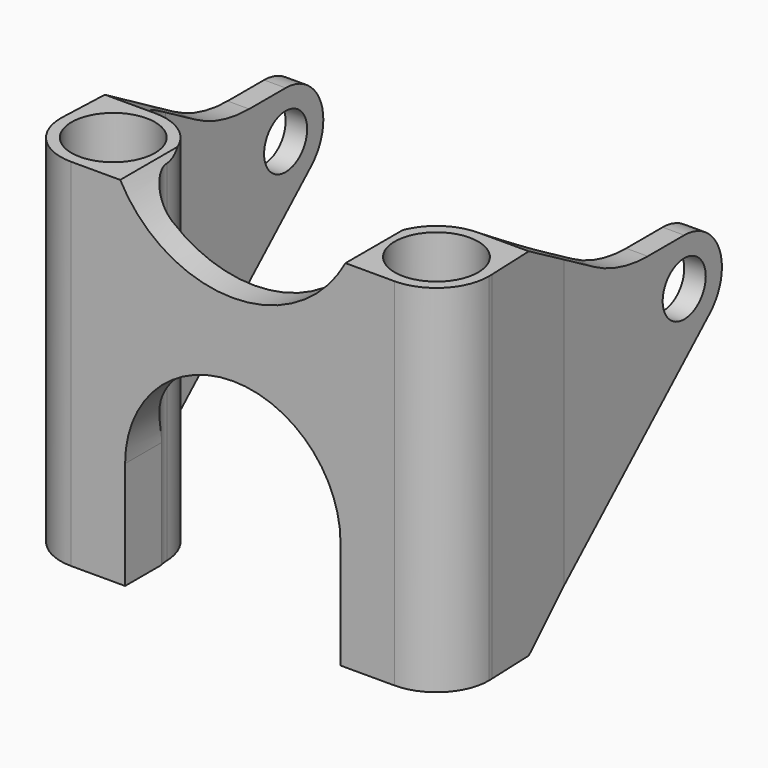
from build123d import *

# Parameters (mm, degrees)
F0_R          = 3.1
F1_DEPTH      = 35
F2_R          = 2
F3_DEPTH      = 31.501
F3_DEPTH_BACK = 0.301
F5_DEPTH      = 25.901


# Not quite as in the source:
# - a feature names something its author has since deleted; it is built from what else it names


with BuildPart() as f1:
    # F0 (on Top) → F1 (new body)
    with BuildSketch(Plane.XY):
        with BuildLine():
            ThreePointArc((-27.9, 0), (-26.7577164466, -2.7577164466), (-24, -3.9))
            ThreePointArc((-24, -3.9), (-21.2422835534, -2.7577164466), (-20.1, 0))
            ThreePointArc((-20.1, 0), (-21.2422835534, 2.7577164466), (-24, 3.9))
            ThreePointArc((-24, 3.9), (-26.643179735, 2.8676821456), (-27.8870765814, 0.3172312247))
            Line((-27.8870765814, 0.3172312247), (-27.9, 0))
        make_face()
        with Locations((-24, 0)):
            Circle(F0_R, mode=Mode.SUBTRACT)
        with BuildLine():
            Line((-27.6, 7.3641016151), (-27.8870765814, 0.3172312247))
            ThreePointArc((-27.8870765814, 0.3172312247), (-26.643179735, 2.8676821456), (-24, 3.9))
            ThreePointArc((-24, 3.9), (-25.4641016151, 5.3641016151), (-26, 7.3641016151))
            Line((-26, 7.3641016151), (-26, 22))
            Line((-26, 22), (-27.6, 22))
            Line((-27.6, 22), (-27.6, 7.3641016151))
        make_face()
        with BuildLine():
            ThreePointArc((0, -3.9), (-2.7577164466, -2.7577164466), (-3.9, 0))
            Line((-3.9, 0), (-3.9, 0.1))
            ThreePointArc((-3.9, 0.1), (-4.4857864376, -1.3142135624), (-5.9, -1.9))
            Line((-5.9, -1.9), (-18.1, -1.9))
            ThreePointArc((-18.1, -1.9), (-19.5142135624, -1.3142135624), (-20.1, 0.1))
            Line((-20.1, 0.1), (-20.1, 0))
            ThreePointArc((-20.1, 0), (-21.2422835534, -2.7577164466), (-24, -3.9))
            Line((-24, -3.9), (0, -3.9))
        make_face()
        with BuildLine():
            Line((3.9, 0), (3.8870765814, 0.3172312247))
            ThreePointArc((3.8870765814, 0.3172312247), (2.643179735, 2.8676821456), (0, 3.9))
            ThreePointArc((0, 3.9), (-2.7577164466, 2.7577164466), (-3.9, 0))
            ThreePointArc((-3.9, 0), (-2.7577164466, -2.7577164466), (0, -3.9))
            ThreePointArc((0, -3.9), (2.7577164466, -2.7577164466), (3.9, 0))
        make_face()
        Circle(F0_R, mode=Mode.SUBTRACT)
        with BuildLine():
            Line((3.6, 7.3641016151), (3.6, 22))
            Line((3.6, 22), (2, 22))
            Line((2, 22), (2, 7.3641016151))
            ThreePointArc((2, 7.3641016151), (1.4641016151, 5.3641016151), (0, 3.9))
            ThreePointArc((0, 3.9), (2.643179735, 2.8676821456), (3.8870765814, 0.3172312247))
            Line((3.8870765814, 0.3172312247), (3.6, 7.3641016151))
        make_face()
    extrude(amount=F1_DEPTH)

    # F2 (on face) → F3 (cut, two sides)
    with BuildSketch(Plane.YZ.offset(3.6)) as f3_sk:
        with BuildLine():
            ThreePointArc((18.5, 21.5), (20.9748737342, 20.4748737342), (22, 18))
            Line((22, 18), (22, 35))
            Line((22, 35), (7.3641016151, 35))
            Line((7.3641016151, 35), (7.3641016151, 24.4293139302))
            Line((7.3641016151, 24.4293139302), (10.1173140978, 22.8397459622))
            ThreePointArc((10.1173140978, 22.8397459622), (12.5291236468, 21.8407417371), (15.1173140978, 21.5))
            Line((15.1173140978, 21.5), (18.5, 21.5))
        make_face()
        Polygon((22, 35), (22, 18), (29.6666024476, 18), (29.6666024476, 42.8468726724), (-4.3945980379, 42.8468726724), (-4.3945980379, 31.2182023401), (7.3641016151, 24.4293139302), (7.3641016151, 35), align=None)
        with Locations((18.5, 18)):
            Circle(F2_R)
        with BuildLine():
            Line((22, 0), (22, 18))
            ThreePointArc((22, 18), (21.7007350945, 16.5839156612), (20.8541172259, 15.4099938057))
            Line((20.8541172259, 15.4099938057), (7.3641016151, 3.1486030042))
            Line((7.3641016151, 3.1486030042), (7.3641016151, 0))
            Line((7.3641016151, 0), (22, 0))
        make_face()
        Polygon((7.3641016151, 0), (7.3641016151, 3.1486030042), (3.9, 0), align=None)
    extrude(amount=-F3_DEPTH, mode=Mode.SUBTRACT)
    extrude(f3_sk.sketch, amount=F3_DEPTH_BACK, mode=Mode.SUBTRACT)

    # F4 (on face) → F5 (cut, through all)
    with BuildSketch(Plane.XZ.offset(3.9)):
        with BuildLine():
            ThreePointArc((-12, 0), (-6.3431457505, 2.3431457505), (-4, 8))
            ThreePointArc((-4, 8), (-12, 16), (-20, 8))
            ThreePointArc((-20, 8), (-17.6568542495, 2.3431457505), (-12, 0))
        make_face()
        with BuildLine():
            Line((-4, 0), (-4, 8))
            ThreePointArc((-4, 8), (-6.3431457505, 2.3431457505), (-12, 0))
            Line((-12, 0), (-4, 0))
        make_face()
        with BuildLine():
            ThreePointArc((-12, 0), (-17.6568542495, 2.3431457505), (-20, 8))
            Line((-20, 8), (-20, 0))
            Line((-20, 0), (-12, 0))
        make_face()
        with BuildLine():
            Line((0, 30.9326460298), (0, 26.4293139302))
            Line((0, 26.4293139302), (8.4664272144, 26.4293139302))
            Line((8.4664272144, 26.4293139302), (8.4664272144, 34.5878303051))
            Line((8.4664272144, 34.5878303051), (-3.2313269012, 34.5878303051))
            ThreePointArc((-3.2313269012, 34.5878303051), (-2.6846257606, 32.7964600712), (-2.5, 30.9326460298))
            Line((-2.5, 30.9326460298), (0, 30.9326460298))
        make_face()
        with BuildLine():
            Line((-3.6351927697, 26.4293139302), (0, 26.4293139302))
            Line((0, 26.4293139302), (0, 30.9326460298))
            Line((0, 30.9326460298), (-2.5, 30.9326460298))
            ThreePointArc((-2.5, 30.9326460298), (-2.7881687844, 28.6105423164), (-3.6351927697, 26.4293139302))
        make_face()
        with BuildLine():
            Line((-24, 30.9326460298), (-24, 26.4293139302))
            Line((-24, 26.4293139302), (-20.3648072303, 26.4293139302))
            ThreePointArc((-20.3648072303, 26.4293139302), (-21.2118312156, 28.6105423164), (-21.5, 30.9326460298))
            Line((-21.5, 30.9326460298), (-24, 30.9326460298))
        make_face()
        with BuildLine():
            Line((-31.3403680921, 26.4293139302), (-24, 26.4293139302))
            Line((-24, 26.4293139302), (-24, 30.9326460298))
            Line((-24, 30.9326460298), (-21.5, 30.9326460298))
            ThreePointArc((-21.5, 30.9326460298), (-21.3153742394, 32.7964600712), (-20.7686730988, 34.5878303051))
            Line((-20.7686730988, 34.5878303051), (-31.3403680921, 34.5878303051))
            Line((-31.3403680921, 34.5878303051), (-31.3403680921, 26.4293139302))
        make_face()
        with BuildLine():
            Line((-20.3648072303, 26.4293139302), (-3.6351927697, 26.4293139302))
            ThreePointArc((-3.6351927697, 26.4293139302), (-2.7881687844, 28.6105423164), (-2.5, 30.9326460298))
            Line((-2.5, 30.9326460298), (-21.5, 30.9326460298))
            ThreePointArc((-21.5, 30.9326460298), (-21.2118312156, 28.6105423164), (-20.3648072303, 26.4293139302))
        make_face()
        with BuildLine():
            ThreePointArc((-20.3648072303, 26.4293139302), (-12, 21.4326460298), (-3.6351927697, 26.4293139302))
            Line((-3.6351927697, 26.4293139302), (-20.3648072303, 26.4293139302))
        make_face()
    extrude(amount=-F5_DEPTH, mode=Mode.SUBTRACT)


solid = f1.part
